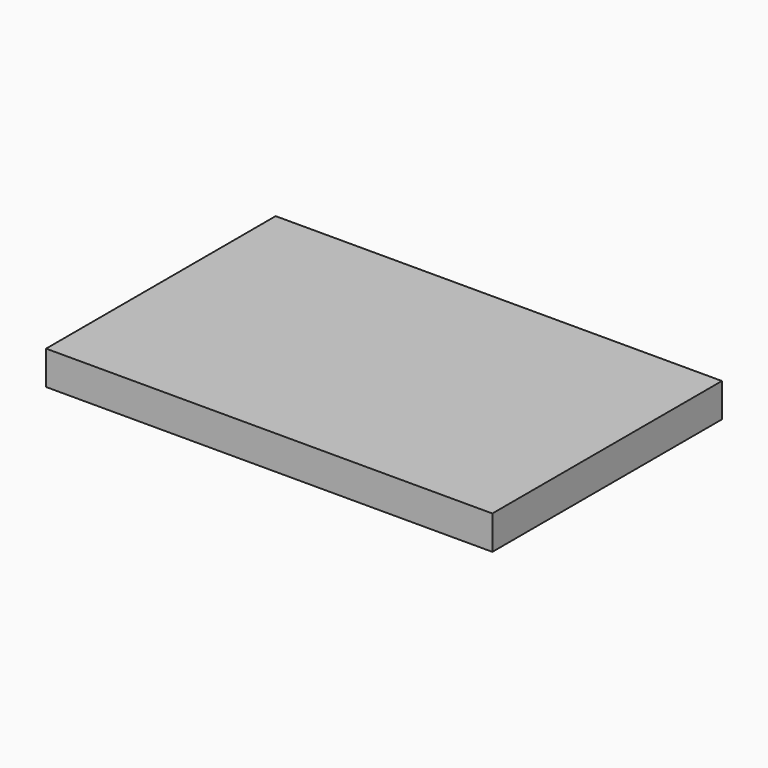
from build123d import *

# Parameters (mm, degrees)
F0_W     = 132.2400420904
F0_H     = 85.026204586
F1_DEPTH = 10.0192911923


# Not quite as in the source:
# - a feature names something its author has since deleted; it is built from what else it names


with BuildPart() as f1:
    # F0 (on Top) → F1 (new body)
    with BuildSketch(Plane.XY):
        Rectangle(F0_W, F0_H)
    extrude(amount=F1_DEPTH)


solid = f1.part
